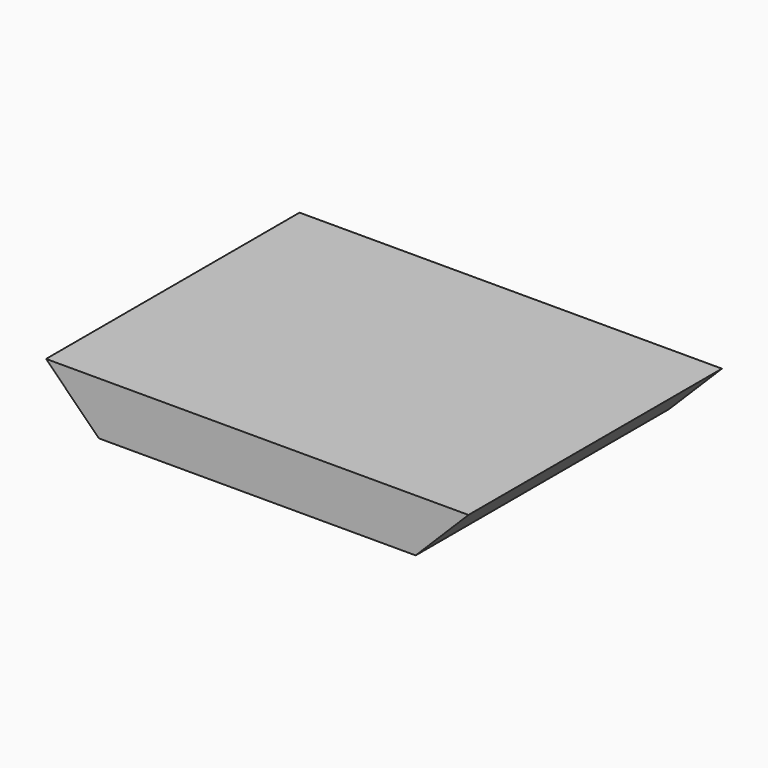
from build123d import *

# Parameters (mm, degrees)
F0_W     = 101.6
F0_H     = 76.2
F1_DEPTH = 12.7
F2_SIZE  = 12.69999


# Not quite as in the source:
# - a fillet or chamfer is up to 0.001 mm smaller than in the source, because OpenCascade refuses the exact size


with BuildPart() as f1:
    # F0 (on Top) → F1 (new body)
    with BuildSketch(Plane.XY):
        with Locations((-3.0236337334, -3.8595628137)):
            Rectangle(F0_W, F0_H)
    extrude(amount=F1_DEPTH)

    # F2 (size 12.7 in the source; OpenCascade refuses exactly that, so slightly less here)
    f2_edges = [f1.edges().sort_by_distance(p)[0] for p in [
        (47.776366, -3.859563, 0),
        (-53.823634, -3.859563, 0),
    ]]
    chamfer(f2_edges, length=F2_SIZE)


solid = f1.part
